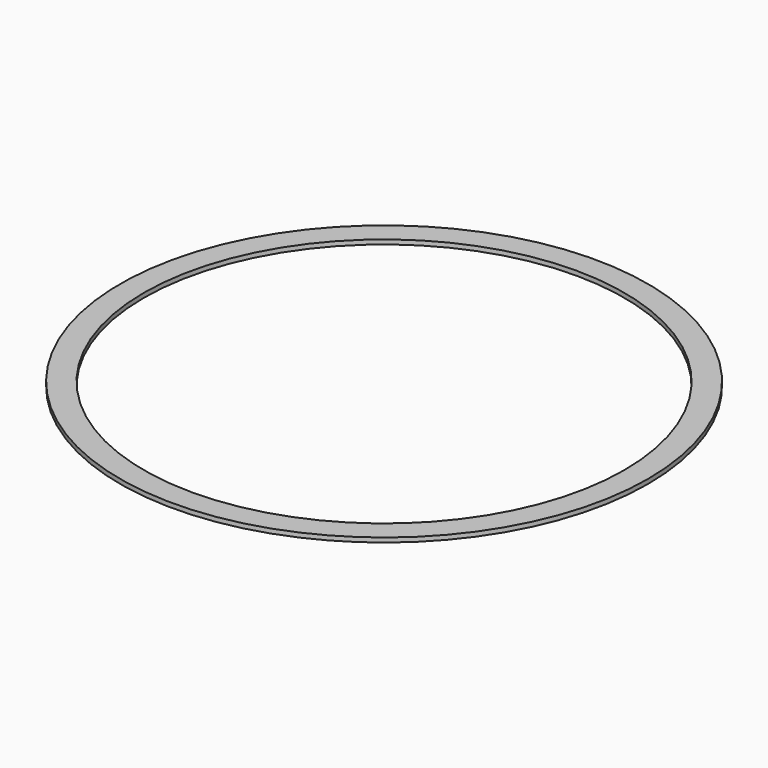
from build123d import *

# Parameters (mm, degrees)
F0_R     = 281.93492
F0_R_2   = 256.53492
F1_DEPTH = 4.7625


# Not quite as in the source:
# - a length typed as a fraction of an inch, garbled in the dataset ("3 / 203.2 mm" for 3/8 in), is restored


with BuildPart() as f1:
    # F0 (on Top) → F1 (new body)
    with BuildSketch(Plane.XY):
        Circle(F0_R)
        Circle(F0_R_2, mode=Mode.SUBTRACT)
    extrude(amount=F1_DEPTH)


solid = f1.part
